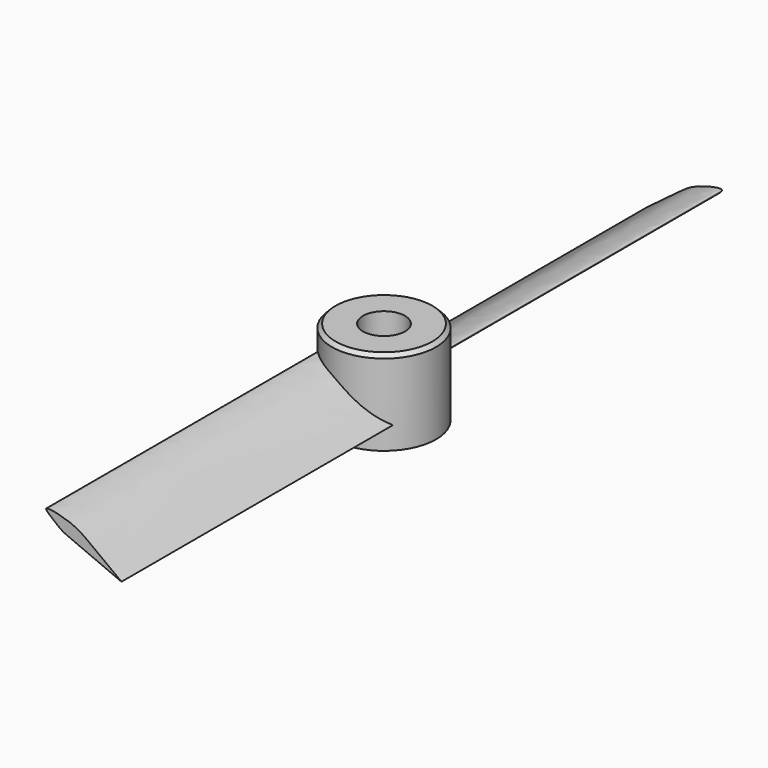
from build123d import *

# Parameters (mm, degrees)
F0_R     = 7.05
F0_R_2   = 2.85
F1_DEPTH = 11.5
F3_DEPTH = 50.8
F4_R     = 5
F6_DEPTH = 50.8
F7_R     = 5
F8_DEPTH = 25
F9_SIZE  = 0.5


# Not quite as in the source:
# - a feature names something its author has since deleted; it is built from what else it names


with BuildPart() as f1:
    # F0 (on Top) → F1 (new body)
    with BuildSketch(Plane.XY):
        Circle(F0_R)
        Circle(F0_R_2, mode=Mode.SUBTRACT)
        Circle(F0_R_2)
    extrude(amount=F1_DEPTH)

    # F2 (on Front) → F3 (join)
    with BuildSketch(Plane.XZ):
        with BuildLine():
            add(Edge.make_bspline(
                [(-3.0257797288, 6.4930361797), (-4.1008577018, 7.46596434), (-6.428713056, 9.0023582287), (-1.9789193009, 8.0350190473), (-0.009488572, 6.9339791337), (2.586277915, 4.8937816415), (4.2564601326, 3.6563219842), (5.0958533903, 3.0405442567)],
                knots=[0, 0, 0, 0, 0.1977876363, 0.3919769243, 0.5835513721, 0.7917756861, 1, 1, 1, 1], degree=3))
            Line((-3.0257797288, 6.4930361797), (5.0958533903, 3.0405442567))
        make_face()
    extrude(amount=F3_DEPTH)

    # F4
    f4_edges = [f1.edges().sort_by_distance(p)[0] for p in [
        (-3.02578, -28.583832, 6.493036),
    ]]
    fillet(f4_edges, radius=F4_R)

    # F5 (on Front) → F6 (join)
    with BuildSketch(Plane.XZ):
        with BuildLine():
            Line((-5.0961042746, 3.0403477398), (3.0255288445, 6.4928396627))
            add(Edge.make_bspline(
                [(3.0255288445, 6.4928396627), (4.1006068175, 7.465767823), (6.4284621717, 9.0021617117), (1.9786684166, 8.0348225303), (0.0092376876, 6.9337826168), (-2.5865287993, 4.8935851245), (-4.2567110169, 3.6561254672), (-5.0961042746, 3.0403477398)],
                knots=[0, 0, 0, 0, 0.1977876363, 0.3919769243, 0.5835513721, 0.7917756861, 1, 1, 1, 1], degree=3))
        make_face()
    extrude(amount=-F6_DEPTH)

    # F7
    f7_edges = [f1.edges().sort_by_distance(p)[0] for p in [
        (3.025529, 28.583892, 6.49284),
    ]]
    fillet(f7_edges, radius=F7_R)

    # F0 (on Top) → F8 (cut)
    with BuildSketch(Plane.XY):
        Circle(F0_R_2)
    extrude(amount=F8_DEPTH, mode=Mode.SUBTRACT)

    # F9
    f9_edges = [f1.edges().sort_by_distance(p)[0] for p in [
        (-7.05, 0, 11.5),
    ]]
    chamfer(f9_edges, length=F9_SIZE)


solid = f1.part
